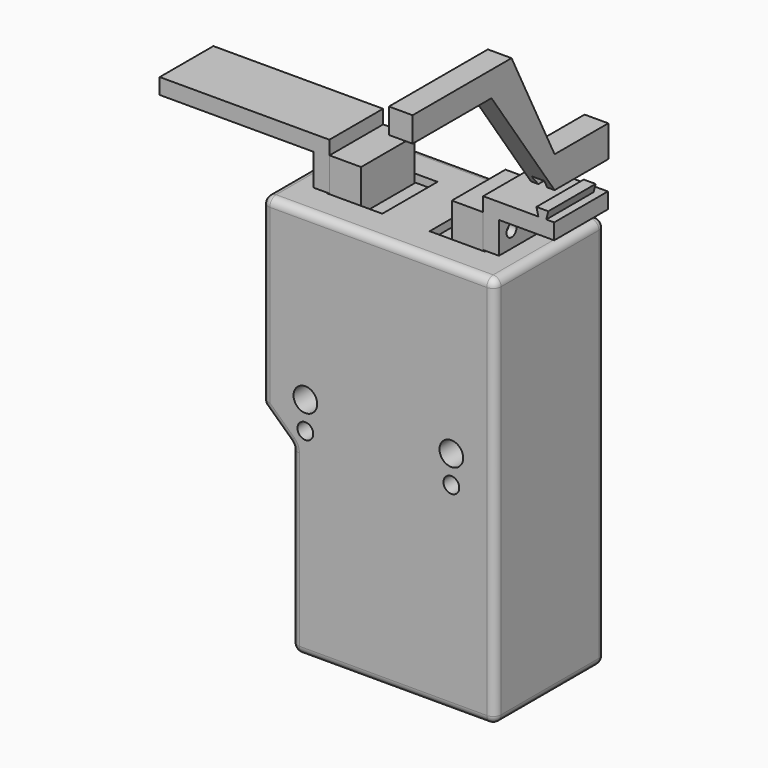
from build123d import *

# Parameters (mm, degrees)
F0_R      = 2
F0_R_2    = 3
F1_DEPTH  = 35
F2_R      = 2
F3_W      = 14
F3_H      = 17.5
F4_DEPTH  = 2
F5_W      = 8
F5_H      = 17
F6_DEPTH  = 10.5
F7_R      = 2
F8_DEPTH  = 2
F9_R      = 2
F10_DEPTH = 2
F12_W     = 17
F12_H     = 12
F12_R     = 1.5875
F13_DEPTH = 4
F14_W     = 17
F14_H     = 4
F15_DEPTH = 18
F17_W     = 17
F17_H     = 12
F17_R     = 1.905
F18_DEPTH = 4
F19_W     = 17
F19_H     = 4
F20_DEPTH = 43
F22_DEPTH = 17
F25_DEPTH = 6
F27_DEPTH = 62.001
F28_W     = 6
F28_H     = 8
F29_DEPTH = 2
F30_W     = 6.4162167525
F30_H     = 2.4192359447
F31_DEPTH = 2


with BuildPart() as f1:
    # F0 (on Front) → F1 (new body)
    with BuildSketch(Plane.XZ):
        with BuildLine():
            ThreePointArc((-2, 0), (-0.5857864376, 0.5857864376), (0, 2))
            Line((0, 2), (0, 97.5))
            ThreePointArc((0, 97.5), (-0.5857864376, 98.9142135624), (-2, 99.5))
            Line((-2, 99.5), (-57, 99.5))
            ThreePointArc((-57, 99.5), (-58.4142135624, 98.9142135624), (-59, 97.5))
            Line((-59, 97.5), (-59, 53.8691046038))
            ThreePointArc((-59, 53.8691046038), (-58.8342945512, 53.0720076842), (-58.3646365007, 52.4069940673))
            Line((-58.3646365007, 52.4069940673), (-52.1353634993, 46.5930059327))
            ThreePointArc((-52.1353634993, 46.5930059327), (-51.6657054488, 45.9279923158), (-51.5, 45.1308953962))
            Line((-51.5, 45.1308953962), (-51.5, 2))
            ThreePointArc((-51.5, 2), (-50.9142135624, 0.5857864376), (-49.5, 0))
            Line((-49.5, 0), (-2, 0))
        make_face()
        with Locations((-48, 50.5)):
            Circle(F0_R, mode=Mode.SUBTRACT)
        with Locations((-48, 57.5)):
            Circle(F0_R_2, mode=Mode.SUBTRACT)
        with Locations((-11, 50.5)):
            Circle(F0_R, mode=Mode.SUBTRACT)
        with Locations((-11, 57.5)):
            Circle(F0_R_2, mode=Mode.SUBTRACT)
    extrude(amount=F1_DEPTH)

    # F2
    f2_edges = [f1.edges().sort_by_distance(p)[0] for p in [
        (0, 0, 49.75),
        (-29.5, -35, 99.5),
        (-51.665705, 0, 45.927992),
        (-51.665705, -35, 45.927992),
        (-51.5, 0, 23.565448),
        (-51.5, -35, 23.565448),
        (-50.914214, 0, 0.585786),
        (-50.914214, -35, 0.585786),
        (-25.75, 0, 0),
        (-25.75, -35, 0),
        (-0.585786, 0, 0.585786),
        (-0.585786, -35, 0.585786),
        (0, -35, 49.75),
        (-0.585786, 0, 98.914214),
        (-0.585786, -35, 98.914214),
        (-29.5, 0, 99.5),
        (-58.414214, 0, 98.914214),
        (-58.414214, -35, 98.914214),
        (-59, 0, 75.684552),
        (-59, -35, 75.684552),
        (-58.834295, 0, 53.072008),
        (-58.834295, -35, 53.072008),
        (-55.25, 0, 49.5),
        (-55.25, -35, 49.5),
    ]]
    fillet(f2_edges, radius=F2_R)

    # F3 (on face) → F4 (cut)
    with BuildSketch(Plane.XY.offset(99.5)):
        with Locations((-42.5, -17.5)):
            Rectangle(F3_W, F3_H)
        with Locations((-16.5, -17.5)):
            Rectangle(F3_W, F3_H)
    extrude(amount=-F4_DEPTH, mode=Mode.SUBTRACT)

    # F5 (on face) → F6 (join)
    with BuildSketch(Plane.XY.offset(97.5)):
        with Locations((-45.0781651735, -17.5)):
            Rectangle(F5_W, F5_H)
        with Locations((-14.0781651735, -17.5)):
            Rectangle(F5_W, F5_H)
    extrude(amount=F6_DEPTH)

    # F7 (on face) → F8 (join)
    with BuildSketch(Plane(origin=(-49.0781651735, 0, 0), x_dir=(0, -1, 0), z_dir=(-1, 0, 0))):
        with Locations((13, 103.5777926445)):
            Circle(F7_R)
        with Locations((22, 103.5777926445)):
            Circle(F7_R)
    extrude(amount=F8_DEPTH)

    # F9 (on face) → F10 (join)
    with BuildSketch(Plane.YZ.offset(-10.0781651735)):
        with Locations((-22, 103.7157326937)):
            Circle(F9_R)
        with Locations((-13, 103.7157326937)):
            Circle(F9_R)
    extrude(amount=F10_DEPTH)


with BuildPart() as f13:
    # F12 (on offset) → F13 (new body)
    with BuildSketch(Plane.YZ.offset(-6.0781651735)):
        with Locations((-17.5719340369, 105.6120348573)):
            Rectangle(F12_W, F12_H)
        with Locations((-22.0719340369, 103.6941558123)):
            Circle(F12_R, mode=Mode.SUBTRACT)
        with Locations((-13.0719340369, 103.6941558123)):
            Circle(F12_R, mode=Mode.SUBTRACT)
    extrude(amount=-F13_DEPTH)

    # F14 (on face) → F15 (join)
    with BuildSketch(Plane(origin=(-10.0781651735, 0, 0), x_dir=(0, -1, 0), z_dir=(-1, 0, 0))):
        with Locations((17.5719340369, 109.6120348573)):
            Rectangle(F14_W, F14_H)
    extrude(amount=-F15_DEPTH)

    # F21 (on face) → F22 (join, through all)
    with BuildSketch(Plane.XZ.offset(26.0719340369)):
        Polygon((3.4218348265, 113.6120348573), (3.9218348265, 111.6120348573), (5.9218348265, 111.6120348573), (6.4218348265, 113.6120348573), align=None)
    extrude(amount=-F22_DEPTH)

    # F30 (on face) → F31 (cut)
    with BuildSketch(Plane(origin=(0, -9.0719340369, 0), x_dir=(-1, 0, 0), z_dir=(0, 1, 0))):
        with Locations((-4.7137264502, 112.8216528296)):
            Rectangle(F30_W, F30_H)
    extrude(amount=-F31_DEPTH, mode=Mode.SUBTRACT)


with BuildPart() as f18:
    # F17 (on offset) → F18 (new body)
    with BuildSketch(Plane(origin=(-53.0781651735, 0, 0), x_dir=(0, -1, 0), z_dir=(-1, 0, 0))):
        with Locations((17.5389906317, 105.5109703541)):
            Rectangle(F17_W, F17_H)
        with Locations((13.0389906317, 103.5974174738)):
            Circle(F17_R, mode=Mode.SUBTRACT)
        with Locations((22.0389906317, 103.5974174738)):
            Circle(F17_R, mode=Mode.SUBTRACT)
    extrude(amount=-F18_DEPTH)

    # F19 (on face) → F20 (join)
    with BuildSketch(Plane.YZ.offset(-49.0781651735)):
        with Locations((-17.5389906317, 109.5109703541)):
            Rectangle(F19_W, F19_H)
    extrude(amount=-F20_DEPTH)


with BuildPart() as f25:
    # F24 (on offset) → F25 (new body)
    with BuildSketch(Plane.YZ.offset(7.9218348265)):
        Polygon((-45.9342463762, 147.4091031194), (-25.9342463762, 118.7591031194), (-8.9342463762, 118.7591031194), (-8.9342463762, 126.7591031194), (-25.9342463762, 126.7591031194), (-39.5842463762, 153.7591031194), (-70.9342463762, 153.7591031194), (-70.9342463762, 147.4091031194), align=None)
    extrude(amount=-F25_DEPTH)

    # F26 (on face) → F27 (cut, through all)
    with BuildSketch(Plane(origin=(0, -8.9342463762, 0), x_dir=(-1, 0, 0), z_dir=(0, 1, 0))):
        Polygon((-6.5468348265, 121.0091031194), (-6.0468348265, 118.7591031194), (-3.7968348265, 118.7591031194), (-3.2968348265, 121.0091031194), align=None)
    extrude(amount=-F27_DEPTH, mode=Mode.SUBTRACT)

    # F28 (on face) → F29 (join)
    with BuildSketch(Plane(origin=(0, -8.9342463762, 0), x_dir=(-1, 0, 0), z_dir=(0, 1, 0))):
        with Locations((-4.9218348265, 122.7591031194)):
            Rectangle(F28_W, F28_H)
    extrude(amount=-F29_DEPTH)


solid = Compound([f1.part, f13.part, f18.part, f25.part])
